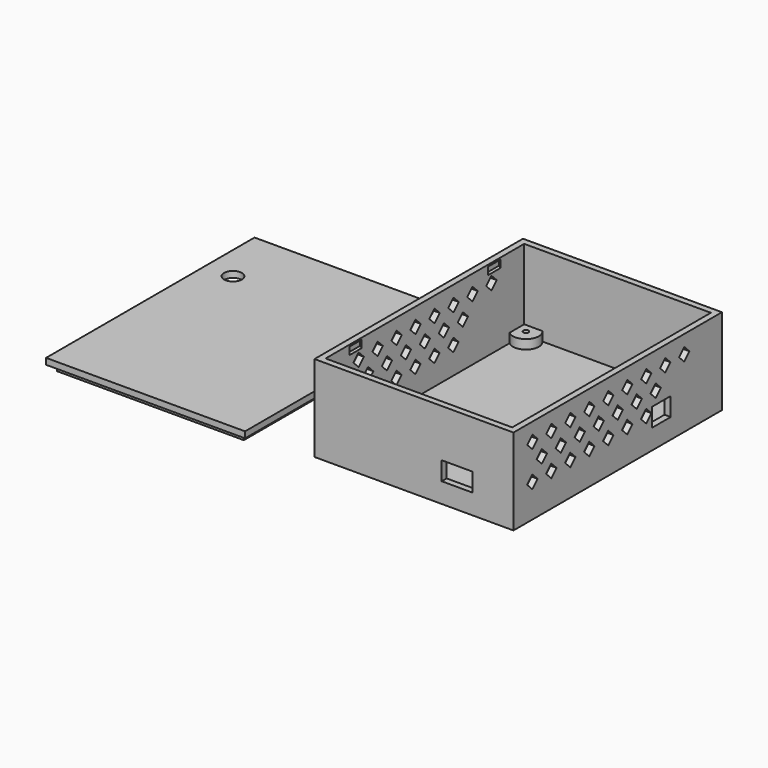
from build123d import *

# Parameters (mm, degrees)
F0_W      = 56.6
F0_H      = 76.6
F1_DEPTH  = 4
F0_R      = 2.9
F0_W_2    = 0.5
F0_H_2    = 5
F2_DEPTH  = 2
F3_START  = -3
F3_DEPTH  = 1
F0_R_2    = 0.85
F4_DEPTH  = 5
F5_DEPTH  = 2
F0_W_3    = 10
F0_H_3    = 2
F0_W_4    = 2
F0_H_4    = 7.5
F6_DEPTH  = 28
F7_START  = 25
F7_DEPTH  = 2
F8_SIZE   = 0.49999
F8_2_SIZE = 0.49999
F9_START  = 6.5
F9_DEPTH  = 6
F11_DEPTH = 80


# Not quite as in the source:
# - a fillet or chamfer is up to 0.001 mm smaller than in the source, because OpenCascade refuses the exact size


with BuildPart() as f1:
    # F0 (on Top) → F1 (new body)
    with BuildSketch(Plane.XY):
        Polygon((-56.8483162045, 25.6724879146), (-56.8483162045, 30.6724879146), (-56.8483162045, 40.3), (-87.1483162045, 40.3), (-117.4483162045, 40.3), (-117.4483162045, 30.6724879146), (-117.4483162045, 25.6724879146), (-117.4483162045, 0), (-117.4483162045, -25.6724879146), (-117.4483162045, -30.6724879146), (-117.4483162045, -40.3), (-87.1483162045, -40.3), (-56.8483162045, -40.3), (-56.8483162045, -30.6724879146), (-56.8483162045, -25.6724879146), (-56.8483162045, 0), align=None)
        with Locations((-87.1483162045, 0)):
            Rectangle(F0_W, F0_H, mode=Mode.SUBTRACT)
    extrude(amount=-F1_DEPTH)

    # F0 (on Top) → F2 (join)
    with BuildSketch(Plane.XY):
        Polygon((-119.4483162045, 42.3), (-119.4483162045, 0), (-119.4483162045, -42.3), (-87.1483162045, -42.3), (-54.8483162045, -42.3), (-54.8483162045, 0), (-54.8483162045, 42.3), (-87.1483162045, 42.3), align=None)
        Polygon((-56.8483162045, 40.3), (-56.8483162045, 30.6724879146), (-56.3483162045, 30.6724879146), (-56.3483162045, 25.6724879146), (-56.8483162045, 25.6724879146), (-56.8483162045, 0), (-56.8483162045, -25.6724879146), (-56.3483162045, -25.6724879146), (-56.3483162045, -30.6724879146), (-56.8483162045, -30.6724879146), (-56.8483162045, -40.3), (-87.1483162045, -40.3), (-117.4483162045, -40.3), (-117.4483162045, -30.6724879146), (-117.9483162045, -30.6724879146), (-117.9483162045, -25.6724879146), (-117.4483162045, -25.6724879146), (-117.4483162045, 0), (-117.4483162045, 25.6724879146), (-117.9483162045, 25.6724879146), (-117.9483162045, 30.6724879146), (-117.4483162045, 30.6724879146), (-117.4483162045, 40.3), (-87.1483162045, 40.3), align=None, mode=Mode.SUBTRACT)
        with Locations((-87.1483162045, 0)):
            Rectangle(F0_W, F0_H)
        with Locations((-110.4483162045, 22.3)):
            Circle(F0_R, mode=Mode.SUBTRACT)
        with Locations((-117.6983162045, 28.1724879146)):
            Rectangle(F0_W_2, F0_H_2)
        with Locations((-56.5983162045, 28.1724879146)):
            Rectangle(F0_W_2, F0_H_2)
        with Locations((-56.5983162045, -28.1724879146)):
            Rectangle(F0_W_2, F0_H_2)
        with Locations((-117.6983162045, -28.1724879146)):
            Rectangle(F0_W_2, F0_H_2)
    extrude(amount=-F2_DEPTH)

    # F0 (on Top) → F3 (join)
    with BuildSketch(Plane.XY.offset(F3_START)):
        with Locations((-56.5983162045, -28.1724879146)):
            Rectangle(F0_W_2, F0_H_2)
        with Locations((-56.5983162045, 28.1724879146)):
            Rectangle(F0_W_2, F0_H_2)
        with Locations((-117.6983162045, 28.1724879146)):
            Rectangle(F0_W_2, F0_H_2)
        with Locations((-117.6983162045, -28.1724879146)):
            Rectangle(F0_W_2, F0_H_2)
    extrude(amount=-F3_DEPTH)

    # F8#2 (size 0.5 in the source; OpenCascade refuses exactly that, so slightly less here)
    f8_2_edges = [f1.edges().sort_by_distance(p)[0] for p in [
        (-117.448316, -28.172488, -3),
        (-117.948316, -28.172488, -4),
        (-117.948316, 28.172488, -4),
        (-117.448316, 28.172488, -3),
        (-56.348316, 28.172488, -4),
        (-56.848316, 28.172488, -3),
        (-56.848316, -28.172488, -3),
        (-56.348316, -28.172488, -4),
    ]]
    chamfer(f8_2_edges, length=F8_2_SIZE)


with BuildPart() as f4:
    # F0 (on Top) → F4 (new body)
    with BuildSketch(Plane.XY):
        with BuildLine():
            ThreePointArc((-30.3, 34.3617650121), (-24.5260700379, 34.5260700379), (-24.3617650121, 40.3))
            Line((-24.3617650121, 40.3), (-30.3, 40.3))
            Line((-30.3, 40.3), (-30.3, 34.3617650121))
        make_face()
        with Locations((-27.5, 37.5)):
            Circle(F0_R_2, mode=Mode.SUBTRACT)
    extrude(amount=F4_DEPTH)



with BuildPart() as f4b:
    # F0 (on Top) → F4, piece 2 (new body)
    with BuildSketch(Plane.XY):
        with BuildLine():
            ThreePointArc((24.3617650121, 40.3), (24.5260700379, 34.5260700379), (30.3, 34.3617650121))
            Line((30.3, 34.3617650121), (30.3, 40.3))
            Line((30.3, 40.3), (24.3617650121, 40.3))
        make_face()
        with Locations((27.5, 37.5)):
            Circle(F0_R_2, mode=Mode.SUBTRACT)
    extrude(amount=F4_DEPTH)


with BuildPart() as f4c:
    # F0 (on Top) → F4, piece 3 (new body)
    with BuildSketch(Plane.XY):
        with BuildLine():
            ThreePointArc((30.3, -34.3617650121), (24.5260700379, -34.5260700379), (24.3617650121, -40.3))
            Line((24.3617650121, -40.3), (30.3, -40.3))
            Line((30.3, -40.3), (30.3, -34.3617650121))
        make_face()
        with Locations((27.5, -37.5)):
            Circle(F0_R_2, mode=Mode.SUBTRACT)
    extrude(amount=F4_DEPTH)


with BuildPart() as f4d:
    # F0 (on Top) → F4, piece 4 (new body)
    with BuildSketch(Plane.XY):
        with BuildLine():
            Line((-30.3, -40.3), (-24.3617650121, -40.3))
            ThreePointArc((-24.3617650121, -40.3), (-24.5260700379, -34.5260700379), (-30.3, -34.3617650121))
            Line((-30.3, -34.3617650121), (-30.3, -40.3))
        make_face()
        with Locations((-27.5, -37.5)):
            Circle(F0_R_2, mode=Mode.SUBTRACT)
    extrude(amount=F4_DEPTH)


with BuildPart() as f4_1:
    add(f4.part)

    add(f4b.part)  # F5 merges F4b

    add(f4c.part)  # F5 merges F4c

    add(f4d.part)  # F5 merges F4d
    # F0 (on Top) → F5 (join)
    with BuildSketch(Plane.XY):
        with BuildLine():
            Line((0, -40.3), (9, -40.3))
            Line((9, -40.3), (19, -40.3))
            Line((19, -40.3), (24.3617650121, -40.3))
            ThreePointArc((24.3617650121, -40.3), (24.5260700379, -34.5260700379), (30.3, -34.3617650121))
            Line((30.3, -34.3617650121), (30.3, -30.6724879146))
            Line((30.3, -30.6724879146), (30.3, -25.6724879146))
            Line((30.3, -25.6724879146), (30.3, 0))
            Line((30.3, 0), (30.3, 14))
            Line((30.3, 14), (30.3, 21.5))
            Line((30.3, 21.5), (30.3, 25.6724879146))
            Line((30.3, 25.6724879146), (30.3, 30.6724879146))
            Line((30.3, 30.6724879146), (30.3, 34.3617650121))
            ThreePointArc((30.3, 34.3617650121), (24.5260700379, 34.5260700379), (24.3617650121, 40.3))
            Line((24.3617650121, 40.3), (0, 40.3))
            Line((0, 40.3), (-24.3617650121, 40.3))
            ThreePointArc((-24.3617650121, 40.3), (-24.5260700379, 34.5260700379), (-30.3, 34.3617650121))
            Line((-30.3, 34.3617650121), (-30.3, 30.6724879146))
            Line((-30.3, 30.6724879146), (-30.3, 25.6724879146))
            Line((-30.3, 25.6724879146), (-30.3, 0))
            Line((-30.3, 0), (-30.3, -25.6724879146))
            Line((-30.3, -25.6724879146), (-30.3, -30.6724879146))
            Line((-30.3, -30.6724879146), (-30.3, -34.3617650121))
            ThreePointArc((-30.3, -34.3617650121), (-24.5260700379, -34.5260700379), (-24.3617650121, -40.3))
            Line((-24.3617650121, -40.3), (0, -40.3))
        make_face()
    extrude(amount=F5_DEPTH)

    # F0 (on Top) → F6 (join)
    with BuildSketch(Plane.XY):
        with Locations((30.55, -28.1724879146)):
            Rectangle(F0_W_2, F0_H_2)
        Polygon((19, -40.3), (19, -42.3), (32.3, -42.3), (32.3, 0), (32.3, 14), (30.3, 14), (30.3, 0), (30.3, -25.6724879146), (30.8, -25.6724879146), (30.8, -30.6724879146), (30.3, -30.6724879146), (30.3, -34.3617650121), (30.3, -40.3), (24.3617650121, -40.3), align=None)
        with Locations((14, -41.3)):
            Rectangle(F0_W_3, F0_H_3)
        Polygon((-32.3, 42.3), (-32.3, 0), (-32.3, -42.3), (0, -42.3), (9, -42.3), (9, -40.3), (0, -40.3), (-24.3617650121, -40.3), (-30.3, -40.3), (-30.3, -34.3617650121), (-30.3, -30.6724879146), (-30.8, -30.6724879146), (-30.8, -25.6724879146), (-30.3, -25.6724879146), (-30.3, 0), (-30.3, 25.6724879146), (-30.8, 25.6724879146), (-30.8, 30.6724879146), (-30.3, 30.6724879146), (-30.3, 34.3617650121), (-30.3, 40.3), (-24.3617650121, 40.3), (0, 40.3), (24.3617650121, 40.3), (30.3, 40.3), (30.3, 34.3617650121), (30.3, 30.6724879146), (30.8, 30.6724879146), (30.8, 25.6724879146), (30.3, 25.6724879146), (30.3, 21.5), (32.3, 21.5), (32.3, 42.3), (0, 42.3), align=None)
        with Locations((31.3, 17.75)):
            Rectangle(F0_W_4, F0_H_4)
        with Locations((30.55, 28.1724879146)):
            Rectangle(F0_W_2, F0_H_2)
        with Locations((-30.55, -28.1724879146)):
            Rectangle(F0_W_2, F0_H_2)
        with Locations((-30.55, 28.1724879146)):
            Rectangle(F0_W_2, F0_H_2)
    extrude(amount=F6_DEPTH)

    # F0 (on Top) → F7 (cut)
    with BuildSketch(Plane.XY.offset(F7_START)):
        with Locations((-30.55, 28.1724879146)):
            Rectangle(F0_W_2, F0_H_2)
        with Locations((-30.55, -28.1724879146)):
            Rectangle(F0_W_2, F0_H_2)
        with Locations((30.55, -28.1724879146)):
            Rectangle(F0_W_2, F0_H_2)
        with Locations((30.55, 28.1724879146)):
            Rectangle(F0_W_2, F0_H_2)
    extrude(amount=F7_DEPTH, mode=Mode.SUBTRACT)

    # F8 (size 0.5 in the source; OpenCascade refuses exactly that, so slightly less here)
    f8_edges = [f4_1.edges().sort_by_distance(p)[0] for p in [
        (-30.8, 28.172488, 25),
        (-30.3, 28.172488, 27),
        (-30.3, -28.172488, 27),
        (-30.8, -28.172488, 25),
        (30.3, 28.172488, 27),
        (30.8, 28.172488, 25),
        (30.3, -28.172488, 27),
        (30.8, -28.172488, 25),
    ]]
    chamfer(f8_edges, length=F8_SIZE)

    # F0 (on Top) → F9 (cut)
    with BuildSketch(Plane.XY.offset(F9_START)):
        with Locations((14, -41.3)):
            Rectangle(F0_W_3, F0_H_3)
        with Locations((31.3, 17.75)):
            Rectangle(F0_W_4, F0_H_4)
    extrude(amount=F9_DEPTH, mode=Mode.SUBTRACT)

    # F10 (on face) → F11 (cut)
    with BuildSketch(Plane.YZ.offset(32.3)):
        Polygon((27, 20.0672313804), (29.1213203436, 22.188551724), (27, 24.3098720675), (24.8786796564, 22.188551724), align=None)
        Polygon((19.3, 20.0672313804), (21.4213203436, 22.188551724), (19.3, 24.3098720675), (17.1786796564, 22.188551724), align=None)
        Polygon((15.4316535859, 14.3658177185), (17.5529739294, 16.487138062), (15.4316535859, 18.6084584056), (13.3103332423, 16.487138062), align=None)
        Polygon((11.5633071717, 12.9070447436), (9.4419868282, 10.7857244001), (11.5633071717, 8.6644040565), (13.6846275153, 10.7857244001), align=None)
        Polygon((7.7316535859, 18.6084584056), (5.6103332423, 16.487138062), (7.7316535859, 14.3658177185), (9.8529739294, 16.487138062), align=None)
        Polygon((11.6, 20.0672313804), (13.7213203436, 22.188551724), (11.6, 24.3098720675), (9.4786796564, 22.188551724), align=None)
        Polygon((3.9, 20.0672313804), (6.0213203436, 22.188551724), (3.9, 24.3098720675), (1.7786796564, 22.188551724), align=None)
        Polygon((0.0316535859, 18.6084584056), (-2.0896667577, 16.487138062), (0.0316535859, 14.3658177185), (2.1529739294, 16.487138062), align=None)
        Polygon((3.8633071717, 12.9070447436), (1.7419868282, 10.7857244001), (3.8633071717, 8.6644040565), (5.9846275153, 10.7857244001), align=None)
        Polygon((-3.8366928283, 12.9070447436), (-5.9580131718, 10.7857244001), (-3.8366928283, 8.6644040565), (-1.7153724847, 10.7857244001), align=None)
        Polygon((-7.6683464141, 18.6084584056), (-9.7896667577, 16.487138062), (-7.6683464141, 14.3658177185), (-5.5470260706, 16.487138062), align=None)
        Polygon((-3.8, 20.0672313804), (-1.6786796564, 22.188551724), (-3.8, 24.3098720675), (-5.9213203436, 22.188551724), align=None)
        Polygon((-11.5, 20.0672313804), (-9.3786796564, 22.188551724), (-11.5, 24.3098720675), (-13.6213203436, 22.188551724), align=None)
        Polygon((-11.5366928283, 12.9070447436), (-13.6580131718, 10.7857244001), (-11.5366928283, 8.6644040565), (-9.4153724847, 10.7857244001), align=None)
        Polygon((-15.3683464141, 18.6084584056), (-17.4896667577, 16.487138062), (-15.3683464141, 14.3658177185), (-13.2470260706, 16.487138062), align=None)
        Polygon((-19.2, 20.0672313804), (-17.0786796564, 22.188551724), (-19.2, 24.3098720675), (-21.3213203436, 22.188551724), align=None)
        Polygon((-20.9470260706, 16.487138062), (-23.0683464141, 18.6084584056), (-25.1896667577, 16.487138062), (-23.0683464141, 14.3658177185), align=None)
        Polygon((-17.1153724847, 10.7857244001), (-19.2366928283, 12.9070447436), (-21.3580131718, 10.7857244001), (-19.2366928283, 8.6644040565), align=None)
        Polygon((-26.9366928283, 12.9070447436), (-29.0580131718, 10.7857244001), (-26.9366928283, 8.6644040565), (-24.8153724847, 10.7857244001), align=None)
        Polygon((-30.7683464141, 18.6084584056), (-32.8896667577, 16.487138062), (-30.7683464141, 14.3658177185), (-28.6470260706, 16.487138062), align=None)
        Polygon((-26.9, 20.0672313804), (-24.7786796564, 22.188551724), (-26.9, 24.3098720675), (-29.0213203436, 22.188551724), align=None)
        Polygon((-34.6, 20.0672313804), (-32.4786796564, 22.188551724), (-34.6, 24.3098720675), (-36.7213203436, 22.188551724), align=None)
        Polygon((-32.5153724847, 10.7857244001), (-34.6366928283, 12.9070447436), (-36.7580131718, 10.7857244001), (-34.6366928283, 8.6644040565), align=None)
    extrude(amount=-F11_DEPTH, mode=Mode.SUBTRACT)


solid = Compound([f1.part, f4_1.part])
